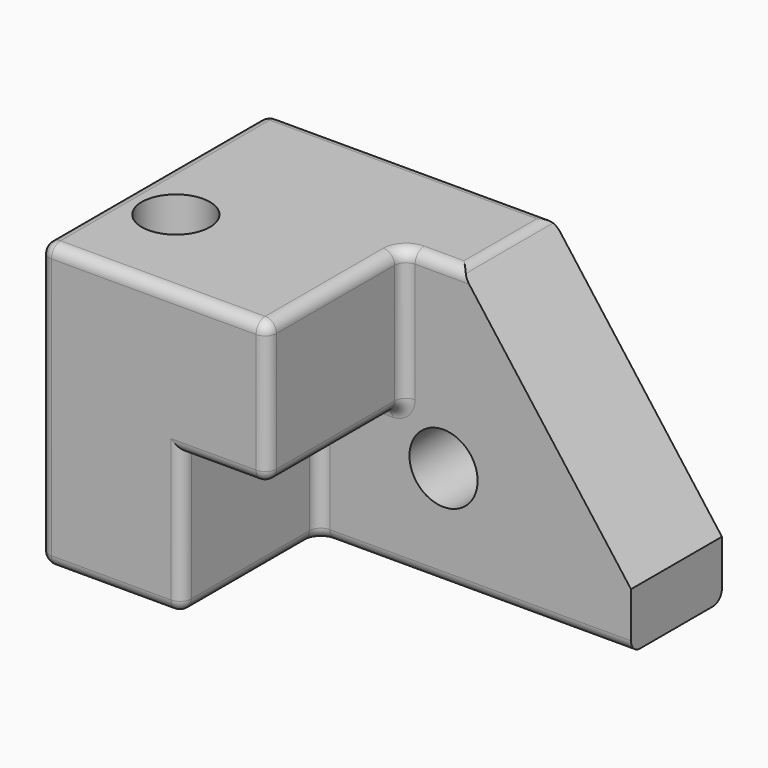
from build123d import *

# Parameters (mm, degrees)
F0_W      = 203.2
F0_H      = 127
F1_DEPTH  = 127
F3_DEPTH  = 76.2
F4_SIZE2  = 101.6
F4_SIZE   = 76.2
F5_R      = 5.08
F6_R      = 15.24
F7_DEPTH  = 50.801
F8_R      = 15.24
F10_DEPTH = 127.001


with BuildPart() as f1:
    # F0 (on Front) → F1 (new body)
    with BuildSketch(Plane.XZ):
        with Locations((2.8009600937, 11.9344207702)):
            Rectangle(F0_W, F0_H)
    extrude(amount=F1_DEPTH)

    # F2 (on face) → F3 (cut)
    with BuildSketch(Plane.XZ.offset(127)):
        Polygon((-35.2990399063, 11.9344207702), (-35.2990399063, -51.5655792298), (104.4009600937, -51.5655792298), (104.4009600937, 75.4344207702), (2.8009600937, 75.4344207702), (2.8009600937, 11.9344207702), align=None)
    extrude(amount=-F3_DEPTH, mode=Mode.SUBTRACT)

    # F4
    f4_edges = [f1.edges().sort_by_distance(p)[0] for p in [
        (104.40096, -25.4, 75.434421),
    ]]
    f4_side = f1.faces().sort_by_distance((-18.970468, -52.614286, 75.434421))[0]
    chamfer(f4_edges, length=F4_SIZE, length2=F4_SIZE2, reference=f4_side)

    # F5
    f5_edges = [f1.edges().sort_by_distance(p)[0] for p in [
        (-47.99904, -127, 75.434421),
        (-98.79904, -63.5, 75.434421),
        (-35.29904, 0, 75.434421),
        (2.80096, -88.9, 75.434421),
        (15.50096, -50.8, 75.434421),
        (2.80096, -50.8, 43.684421),
        (2.80096, -127, 43.684421),
        (2.80096, -88.9, 11.934421),
        (-35.29904, -50.8, -19.815579),
        (34.55096, -50.8, -51.565579),
        (-35.29904, -88.9, -51.565579),
        (-35.29904, -127, -19.815579),
        (-67.04904, -127, -51.565579),
        (-98.79904, -127, 11.934421),
        (2.80096, 0, -51.565579),
        (-98.79904, 0, 11.934421),
        (-98.79904, -63.5, -51.565579),
        (28.20096, -25.4, 75.434421),
        (-16.24904, -127, 11.934421),
        (-16.24904, -50.8, 11.934421),
    ]]
    fillet(f5_edges, radius=F5_R)

    # F6 (on face) → F7 (cut, through all)
    with BuildSketch(Plane.XZ.offset(50.8)):
        with Locations((20.5809600937, -5.8455792298)):
            Circle(F6_R)
    extrude(amount=-F7_DEPTH, mode=Mode.SUBTRACT)

    # F8 (on face) → F10 (cut, through all)
    with BuildSketch(Plane.XY.offset(75.4344207702)):
        with Locations((-74.706427753, -81.28)):
            Circle(F8_R)
    extrude(amount=-F10_DEPTH, mode=Mode.SUBTRACT)


solid = f1.part
